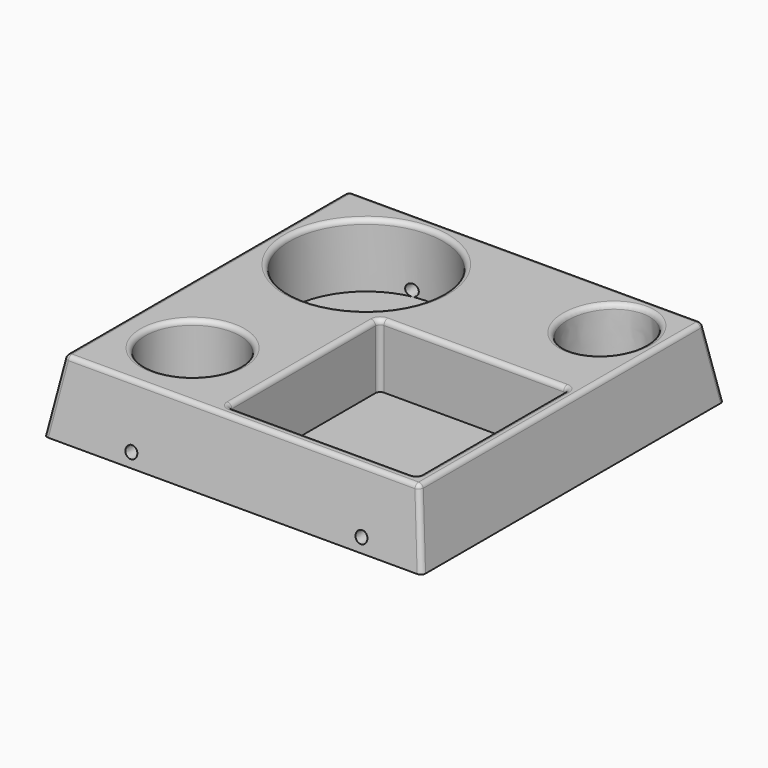
from build123d import *

# Parameters (mm, degrees)
F2_W     = 150.0000023842
F2_H     = 150.0000023842
F0_W     = 160
F0_H     = 160
F4_R     = 32.5
F4_R_2   = 20
F4_W     = 80
F4_H     = 80
F5_DEPTH = 27
F8_DEPTH = 160.0010001
F10_R    = 2


# Not quite as in the source:
# - a feature of the source that left no trace in its solid (it failed there, or was rolled back) is left out


with BuildPart() as f3:
    # F2 (on offset) → F3 section 0
    with BuildSketch(Plane.XY.offset(30)):
        with Locations((80, 80)):
            Rectangle(F2_W, F2_H)
    # F0 (on Top) → F3 section 1
    with BuildSketch(Plane.XY):
        with Locations((80, 80)):
            Rectangle(F0_W, F0_H)
    loft()

    # F4 (on face) → F5 (cut)
    with BuildSketch(Plane.XY.offset(30)):
        with Locations((42.4999988079, 117.5000011921)):
            Circle(F4_R)
        with Locations((34.9999988079, 34.9999988079)):
            Circle(F4_R_2)
        with Locations((110.0000011921, 49.9999988079)):
            Rectangle(F4_W, F4_H)
        with BuildLine():
            add(Edge.make_bspline(
                [(133.5000011921, 112.0000011921), (162.078839517, 112.0000011921), (147.7894203545, 140.5000011921), (133.5000011921, 169.0000011921), (119.2105820296, 140.5000011921), (104.9211628672, 112.0000011921), (133.5000011921, 112.0000011921)],
                knots=[0, 0, 0, 2.0943951024, 2.0943951024, 4.1887902048, 4.1887902048, 6.2831853072, 6.2831853072, 6.2831853072], degree=2, weights=[1, 0.5, 1, 0.5, 1, 0.5, 1]))
        make_face()
    extrude(amount=-F5_DEPTH, mode=Mode.SUBTRACT)

    # F7 (on Front) → F8 (cut, through all)
    with BuildSketch(Plane.XZ):
        with BuildLine():
            add(Edge.make_bspline(
                [(136.252822496, 5.4695543429), (136.252822496, 9.7407653513), (132.502822496, 7.6051598471), (128.752822496, 5.4695543429), (132.502822496, 3.3339488387), (136.252822496, 1.1983433345), (136.252822496, 5.4695543429)],
                knots=[0, 0, 0, 2.0943951024, 2.0943951024, 4.1887902048, 4.1887902048, 6.2831853072, 6.2831853072, 6.2831853072], degree=2, weights=[1, 0.5, 1, 0.5, 1, 0.5, 1]))
        make_face()
        with BuildLine():
            add(Edge.make_bspline(
                [(38.8814116363, 5.4695543429), (38.8814116363, 9.7407653513), (35.1314116363, 7.6051598471), (31.3814116363, 5.4695543429), (35.1314116363, 3.3339488387), (38.8814116363, 1.1983433345), (38.8814116363, 5.4695543429)],
                knots=[0, 0, 0, 2.0943951024, 2.0943951024, 4.1887902048, 4.1887902048, 6.2831853072, 6.2831853072, 6.2831853072], degree=2, weights=[1, 0.5, 1, 0.5, 1, 0.5, 1]))
        make_face()
    extrude(amount=-F8_DEPTH, mode=Mode.SUBTRACT)

    # F10
    f10_edges = [f3.edges().sort_by_distance(p)[0] for p in [
        (150.000001, 49.999999, 30),
        (110.000001, 89.999999, 30),
        (150.000001, 89.999999, 16.5),
        (150.000001, 9.999999, 16.5),
        (70.000001, 9.999999, 16.5),
        (70.000001, 89.999999, 16.5),
        (14.999999, 34.999999, 30),
        (9.999999, 117.500001, 30),
        (133.500001, 150.000001, 30),
        (80, 155.000001, 30),
        (80, 4.999999, 30),
        (2.499999, 2.499999, 15),
        (157.500001, 2.499999, 15),
        (4.999999, 80, 30),
        (155.000001, 80, 30),
        (110.000001, 9.999999, 30),
        (70.000001, 49.999999, 30),
        (2.499999, 157.500001, 15),
        (157.500001, 157.500001, 15),
    ]]
    fillet(f10_edges, radius=F10_R)


solid = f3.part
